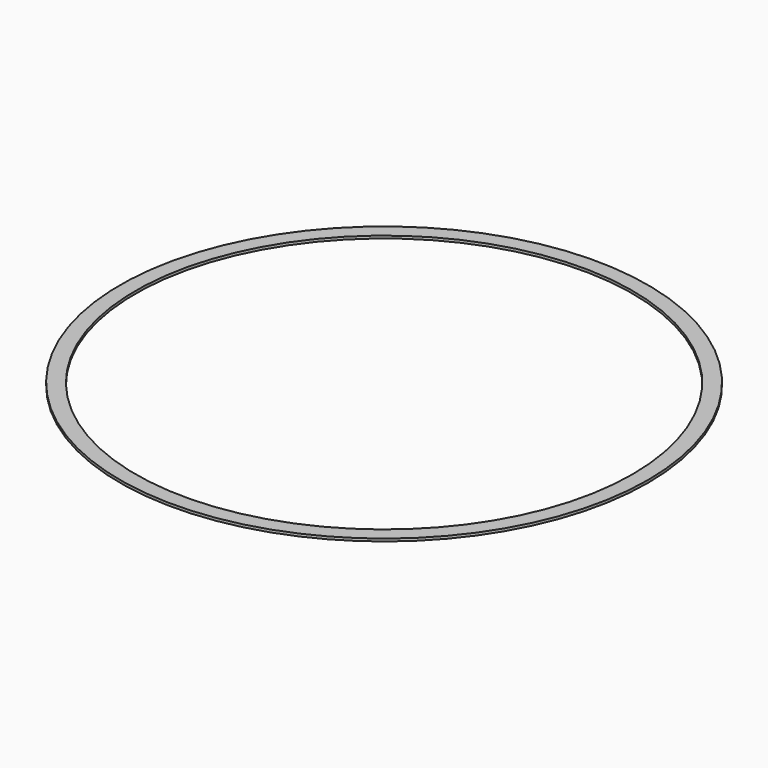
from build123d import *

# Parameters (mm, degrees)
F0_R     = 433.29098
F0_R_2   = 407.89098
F1_DEPTH = 4.2333333333


# Not quite as in the source:
# - a length typed as a fraction of an inch, garbled in the dataset ("3 / 203.2 mm" for 3/8 in), is restored


with BuildPart() as f1:
    # F0 (on Top) → F1 (new body)
    with BuildSketch(Plane.XY):
        Circle(F0_R)
        Circle(F0_R_2, mode=Mode.SUBTRACT)
    extrude(amount=F1_DEPTH)


solid = f1.part
